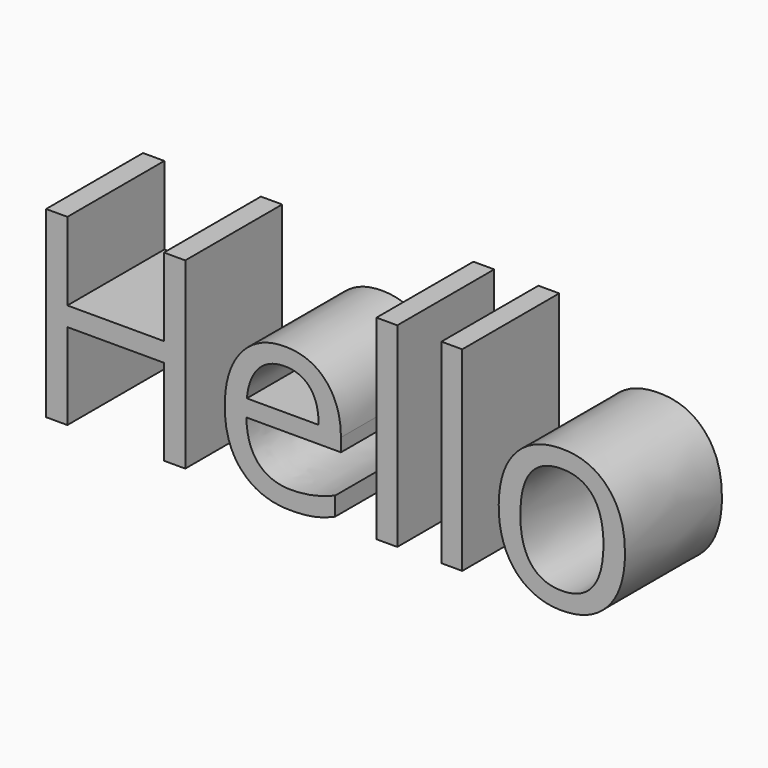
from build123d import *

# Parameters (mm, degrees)
F0_TEXT_SIZE = 53.8198691275
F1_DEPTH     = 25.4


# Not quite as in the source:
# - Text() gives the source's letters only with a copy of the font that has no kerning and outlines rounded to 1/6400 em; it was checked with that copy


with BuildPart() as f1:
    # F0 (on Front) → F1 (new body)
    with BuildSketch(Plane.XZ):
        with Locations((-130.1095336158, -38.7503057718)):
            Text('Hello', F0_TEXT_SIZE, font='Open Sans', text_align=(TextAlign.LEFT, TextAlign.BOTTOM))
    extrude(amount=F1_DEPTH)


solid = f1.part
